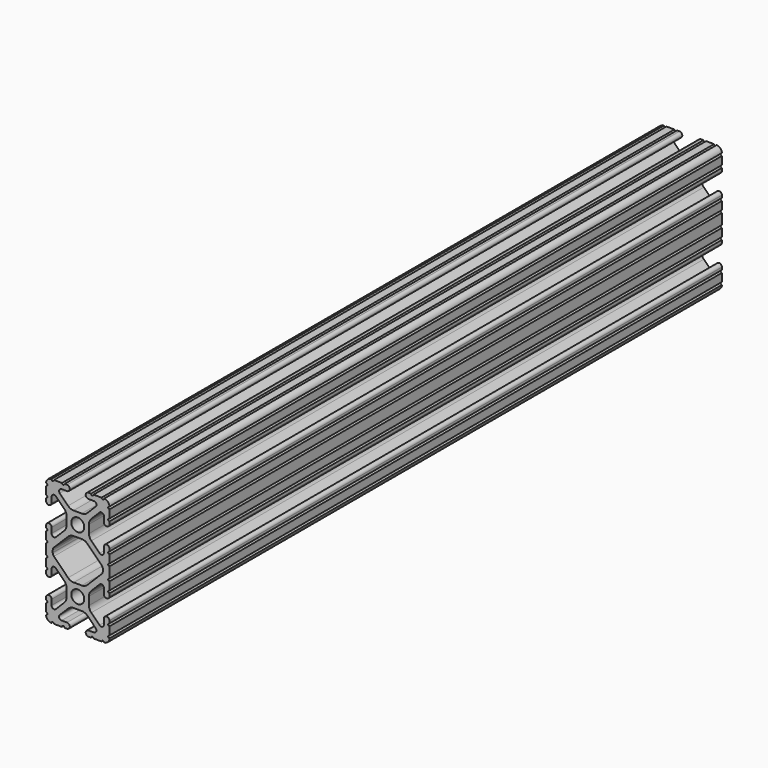
from build123d import *

# Parameters (mm, degrees)
F1_DEPTH = 307


# Not quite as in the source:
# - ends of sketch curves that miss each other by under 0.0002 mm in the source are joined


with BuildPart() as f1:
    # F0 (on Front) → F1 (new body)
    with BuildSketch(Plane.XZ):
        with BuildLine():
            ThreePointArc((-12.6999998568, 23.2791116031), (-12.1919492, 22.76475), (-12.6999998568, 22.2503883969))
            Line((-12.6999998568, 22.2503883969), (-12.7, 19.0246))
            ThreePointArc((-12.7, 19.0246), (-12.192, 18.5166), (-12.7, 18.0086))
            Line((-12.7, 18.0086), (-12.7, 17.0023028))
            ThreePointArc((-12.7, 17.0023028), (-11.5951, 15.8974028), (-10.4902, 17.0023028))
            Line((-10.4902, 17.0023028), (-10.4902, 19.1747902))
            ThreePointArc((-10.4902, 19.1747902), (-9.8630063673, 20.113451805), (-8.7557795103, 19.8932106897))
            Line((-8.7557795103, 19.8932106897), (-5.4384448, 16.5758622))
            ThreePointArc((-5.4384448, 16.5758622), (-4.7501824843, 15.5458268978), (-4.5085, 14.330807))
            Line((-4.5085, 14.330807), (-4.5085, 11.069193))
            ThreePointArc((-4.5085, 11.069193), (-4.7501824843, 9.8541731022), (-5.4384359697, 8.8241289697))
            Line((-5.4384359697, 8.8241289697), (-8.7557864, 5.5067962))
            ThreePointArc((-8.7557864, 5.5067962), (-9.8630063673, 5.286548195), (-10.4902, 6.2252098))
            Line((-10.4902, 6.2252098), (-10.4902, 8.3976972))
            ThreePointArc((-10.4902, 8.3976972), (-11.5951, 9.5025972), (-12.7, 8.3976972))
            Line((-12.7, 8.3976972), (-12.7, 7.3914))
            ThreePointArc((-12.7, 7.3914), (-12.192, 6.8834), (-12.7, 6.3754))
            Line((-12.7, 6.3754), (-12.7, 3.1496))
            ThreePointArc((-12.7, 3.1496), (-12.192, 2.6416), (-12.7, 2.1336))
            Line((-12.7, 2.1336), (-12.7, -2.1336))
            ThreePointArc((-12.7, -2.1336), (-12.192, -2.6416), (-12.7, -3.1496))
            Line((-12.7, -3.1496), (-12.7, -6.3754))
            ThreePointArc((-12.7, -6.3754), (-12.192, -6.8834), (-12.7, -7.3914))
            Line((-12.7, -7.3914), (-12.7, -8.3976972))
            ThreePointArc((-12.7, -8.3976972), (-11.5951, -9.5025972), (-10.4902, -8.3976972))
            Line((-10.4902, -8.3976972), (-10.4902, -6.2252098))
            ThreePointArc((-10.4902, -6.2252098), (-9.8630063673, -5.286548195), (-8.7557795103, -5.5067893103))
            Line((-8.7557795103, -5.5067893103), (-5.4384448, -8.8241378))
            ThreePointArc((-5.4384448, -8.8241378), (-4.7501824843, -9.8541731022), (-4.5085, -11.069193))
            Line((-4.5085, -11.069193), (-4.5085, -14.330807))
            ThreePointArc((-4.5085, -14.330807), (-4.7501824843, -15.5458268978), (-5.4384359697, -16.5758710303))
            Line((-5.4384359697, -16.5758710303), (-8.7557864, -19.8932038))
            ThreePointArc((-8.7557864, -19.8932038), (-9.8630063673, -20.113451805), (-10.4902, -19.1747902))
            Line((-10.4902, -19.1747902), (-10.4902, -17.0023028))
            ThreePointArc((-10.4902, -17.0023028), (-11.5951, -15.8974028), (-12.7, -17.0023028))
            Line((-12.7, -17.0023028), (-12.7, -18.0086))
            ThreePointArc((-12.7, -18.0086), (-12.192, -18.5166), (-12.7, -19.0246))
            Line((-12.7, -19.0246), (-12.7, -22.2504))
            ThreePointArc((-12.7, -22.2504), (-12.1919492, -22.76475), (-12.6999998568, -23.2791116031))
            ThreePointArc((-12.6999998568, -23.2791116031), (-12.0825733161, -24.7825733161), (-10.579099926, -25.4000122396))
            ThreePointArc((-10.579099926, -25.4000122396), (-10.06475, -24.8919492), (-9.5503883969, -25.3999998568))
            Line((-9.5503883969, -25.3999998568), (-6.3246, -25.4))
            ThreePointArc((-6.3246, -25.4), (-5.8166, -24.892), (-5.3086, -25.4))
            Line((-5.3086, -25.4), (-4.3023028, -25.4))
            ThreePointArc((-4.3023028, -25.4), (-3.1974028, -24.2951), (-4.3023028, -23.1902))
            Line((-4.3023028, -23.1902), (-6.4747902, -23.1902))
            ThreePointArc((-6.4747902, -23.1902), (-7.413451805, -22.5630063673), (-7.1932106897, -21.4557795103))
            Line((-7.1932106897, -21.4557795103), (-3.8758622, -18.1384448))
            ThreePointArc((-3.8758622, -18.1384448), (-2.8458268978, -17.4501824843), (-1.630807, -17.2085))
            Line((-1.630807, -17.2085), (1.630807, -17.2085))
            ThreePointArc((1.630807, -17.2085), (2.8458268978, -17.4501824843), (3.8758710303, -18.1384359697))
            Line((3.8758710303, -18.1384359697), (7.1932038, -21.4557864))
            ThreePointArc((7.1932038, -21.4557864), (7.413451805, -22.5630063673), (6.4747902, -23.1902))
            Line((6.4747902, -23.1902), (4.3023028, -23.1902))
            ThreePointArc((4.3023028, -23.1902), (3.1974028, -24.2951), (4.3023028, -25.4))
            Line((4.3023028, -25.4), (5.3086, -25.4))
            ThreePointArc((5.3086, -25.4), (5.8166, -24.892), (6.3246, -25.4))
            Line((6.3246, -25.4), (9.5504, -25.4))
            ThreePointArc((9.5504, -25.4), (10.06475, -24.8919492), (10.5791116031, -25.3999998568))
            ThreePointArc((10.5791116031, -25.3999998568), (12.0825733161, -24.7825733161), (12.7000122396, -23.279099926))
            ThreePointArc((12.7000122396, -23.279099926), (12.1919492, -22.76475), (12.6999998568, -22.2503883969))
            Line((12.6999998568, -22.2503883969), (12.7, -19.0246))
            ThreePointArc((12.7, -19.0246), (12.192, -18.5166), (12.7, -18.0086))
            Line((12.7, -18.0086), (12.7, -17.0023028))
            ThreePointArc((12.7, -17.0023028), (11.5951, -15.8974028), (10.4902, -17.0023028))
            Line((10.4902, -17.0023028), (10.4902, -19.1747902))
            ThreePointArc((10.4902, -19.1747902), (9.8630063673, -20.113451805), (8.7557795103, -19.8932106897))
            Line((8.7557795103, -19.8932106897), (5.4384448, -16.5758622))
            ThreePointArc((5.4384448, -16.5758622), (4.7501824843, -15.5458268978), (4.5085, -14.330807))
            Line((4.5085, -14.330807), (4.5085, -11.069193))
            ThreePointArc((4.5085, -11.069193), (4.7501824843, -9.8541731022), (5.4384359697, -8.8241289697))
            Line((5.4384359697, -8.8241289697), (8.7557864, -5.5067962))
            ThreePointArc((8.7557864, -5.5067962), (9.8630063673, -5.286548195), (10.4902, -6.2252098))
            Line((10.4902, -6.2252098), (10.4902, -8.3976972))
            ThreePointArc((10.4902, -8.3976972), (11.5951, -9.5025972), (12.7, -8.3976972))
            Line((12.7, -8.3976972), (12.7, -7.3914))
            ThreePointArc((12.7, -7.3914), (12.192, -6.8834), (12.7, -6.3754))
            Line((12.7, -6.3754), (12.7, -3.1496))
            ThreePointArc((12.7, -3.1496), (12.192, -2.6416), (12.7, -2.1336))
            Line((12.7, -2.1336), (12.7, 2.1336))
            ThreePointArc((12.7, 2.1336), (12.192, 2.6416), (12.7, 3.1496))
            Line((12.7, 3.1496), (12.7, 6.3754))
            ThreePointArc((12.7, 6.3754), (12.192, 6.8834), (12.7, 7.3914))
            Line((12.7, 7.3914), (12.7, 8.3976972))
            ThreePointArc((12.7, 8.3976972), (11.5951, 9.5025972), (10.4902, 8.3976972))
            Line((10.4902, 8.3976972), (10.4902, 6.2252098))
            ThreePointArc((10.4902, 6.2252098), (9.8630063673, 5.286548195), (8.7557795103, 5.5067893103))
            Line((8.7557795103, 5.5067893103), (5.4384448, 8.8241378))
            ThreePointArc((5.4384448, 8.8241378), (4.7501824843, 9.8541731022), (4.5085, 11.069193))
            Line((4.5085, 11.069193), (4.5085, 14.330807))
            ThreePointArc((4.5085, 14.330807), (4.7501824843, 15.5458268978), (5.4384359697, 16.5758710303))
            Line((5.4384359697, 16.5758710303), (8.7557864, 19.8932038))
            ThreePointArc((8.7557864, 19.8932038), (9.8630063673, 20.113451805), (10.4902, 19.1747902))
            Line((10.4902, 19.1747902), (10.4902, 17.0023028))
            ThreePointArc((10.4902, 17.0023028), (11.5951, 15.8974028), (12.7, 17.0023028))
            Line((12.7, 17.0023028), (12.7, 18.0086))
            ThreePointArc((12.7, 18.0086), (12.192, 18.5166), (12.7, 19.0246))
            Line((12.7, 19.0246), (12.7, 22.2504))
            ThreePointArc((12.7, 22.2504), (12.1919492, 22.76475), (12.6999998568, 23.2791116031))
            ThreePointArc((12.6999998568, 23.2791116031), (12.0825733161, 24.7825733161), (10.579099926, 25.4000122396))
            ThreePointArc((10.579099926, 25.4000122396), (10.06475, 24.8919492), (9.5503883969, 25.3999998568))
            Line((9.5503883969, 25.3999998568), (6.3246, 25.4))
            ThreePointArc((6.3246, 25.4), (5.8166, 24.892), (5.3086, 25.4))
            Line((5.3086, 25.4), (4.3023028, 25.4))
            ThreePointArc((4.3023028, 25.4), (3.1974028, 24.2951), (4.3023028, 23.1902))
            Line((4.3023028, 23.1902), (6.4747902, 23.1902))
            ThreePointArc((6.4747902, 23.1902), (7.413451805, 22.5630063673), (7.1932106897, 21.4557795103))
            Line((7.1932106897, 21.4557795103), (3.8758622, 18.1384448))
            ThreePointArc((3.8758622, 18.1384448), (2.8458268978, 17.4501824843), (1.630807, 17.2085))
            Line((1.630807, 17.2085), (-1.630807, 17.2085))
            ThreePointArc((-1.630807, 17.2085), (-2.8458268978, 17.4501824843), (-3.8758710303, 18.1384359697))
            Line((-3.8758710303, 18.1384359697), (-7.1932038, 21.4557864))
            ThreePointArc((-7.1932038, 21.4557864), (-7.413451805, 22.5630063673), (-6.4747902, 23.1902))
            Line((-6.4747902, 23.1902), (-4.3023028, 23.1902))
            ThreePointArc((-4.3023028, 23.1902), (-3.1974028, 24.2951), (-4.3023028, 25.4))
            Line((-4.3023028, 25.4), (-5.3086, 25.4))
            ThreePointArc((-5.3086, 25.4), (-5.8166, 24.892), (-6.3246, 25.4))
            Line((-6.3246, 25.4), (-9.5504, 25.4))
            ThreePointArc((-9.5504, 25.4), (-10.06475, 24.8919492), (-10.5791116031, 25.3999998568))
            ThreePointArc((-10.5791116031, 25.3999998568), (-12.0825733161, 24.7825733161), (-12.6999998568, 23.2791116031))
        make_face()
        with BuildLine():
            ThreePointArc((-2.6035, -12.7), (0, -10.0965), (2.6035, -12.7))
            ThreePointArc((2.6035, -12.7), (0, -15.3035), (-2.6035, -12.7))
        make_face(mode=Mode.SUBTRACT)
        with BuildLine():
            ThreePointArc((-10.033, 0.45212), (-9.9131254878, 1.0547698693), (-9.571751759, 1.565671759))
            Line((-9.571751759, 1.565671759), (-3.8758622, 7.2615552))
            ThreePointArc((-3.8758622, 7.2615552), (-2.8458268978, 7.9498175157), (-1.630807, 8.1915))
            Line((-1.630807, 8.1915), (1.630807, 8.1915))
            ThreePointArc((1.630807, 8.1915), (2.8458268978, 7.9498175157), (3.8758710303, 7.2615640303))
            Line((3.8758710303, 7.2615640303), (9.5717614, 1.5656814))
            ThreePointArc((9.5717614, 1.5656814), (9.9131254878, 1.0547698693), (10.033, 0.45212))
            Line((10.033, 0.45212), (10.033, -0.45212))
            ThreePointArc((10.033, -0.45212), (9.9131254878, -1.0547698693), (9.571751759, -1.565671759))
            Line((9.571751759, -1.565671759), (3.8758622, -7.2615552))
            ThreePointArc((3.8758622, -7.2615552), (2.8458268978, -7.9498175157), (1.630807, -8.1915))
            Line((1.630807, -8.1915), (-1.630807, -8.1915))
            ThreePointArc((-1.630807, -8.1915), (-2.8458268978, -7.9498175157), (-3.8758710303, -7.2615640303))
            Line((-3.8758710303, -7.2615640303), (-9.5717614, -1.5656814))
            ThreePointArc((-9.5717614, -1.5656814), (-9.9131254878, -1.0547698693), (-10.033, -0.45212))
            Line((-10.033, -0.45212), (-10.033, 0.45212))
        make_face(mode=Mode.SUBTRACT)
        with BuildLine():
            ThreePointArc((-2.6035, 12.7), (0, 15.3035), (2.6035, 12.7))
            ThreePointArc((2.6035, 12.7), (0, 10.0965), (-2.6035, 12.7))
        make_face(mode=Mode.SUBTRACT)
    extrude(amount=F1_DEPTH)


solid = f1.part
